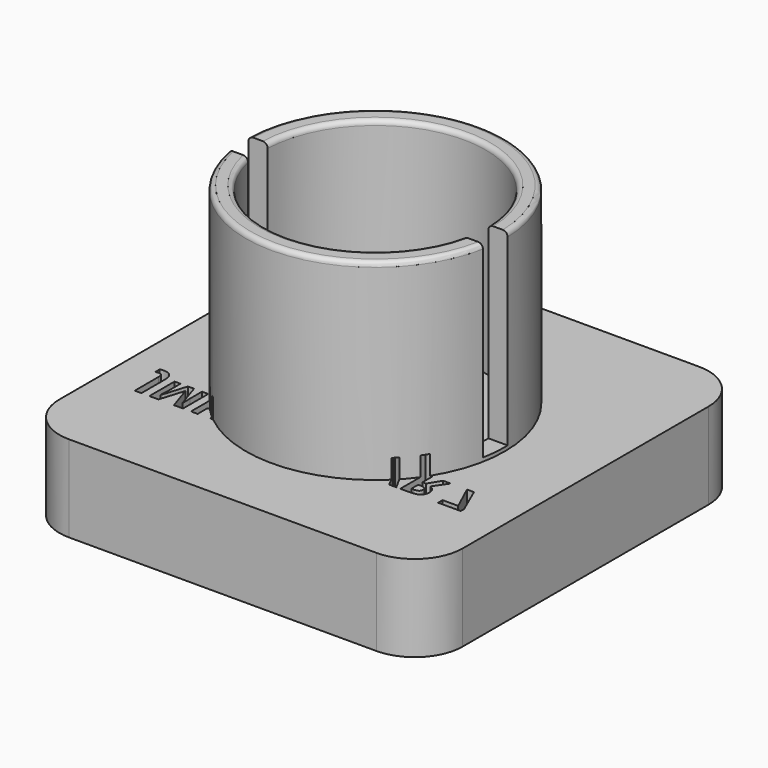
from build123d import *

# Parameters (mm, degrees)
F1_DEPTH      = 3
F2_R          = 13.5
F3_DEPTH      = 20
F4_T          = -2
F5_R          = 0.5
F6_TEXT_SIZE  = 4.5962860367
F7_DEPTH      = 5
F8_W          = 2.9094833881
F8_H          = 24.4396554772
F9_DEPTH      = 61.5
F10_DEPTH     = 6
F11_TEXT_SIZE = 3.6623448817
F12_DEPTH     = 7


# Not quite as in the source:
# - Text() gives the source's letters only with a copy of the font that has no kerning and outlines rounded to 1/6400 em; it was checked with that copy


with BuildPart() as f1:
    # F0 (on Top) → F1 (new body)
    with BuildSketch(Plane.XY):
        with BuildLine():
            ThreePointArc((0, 5), (1.4644660941, 1.4644660941), (5, 0))
            Line((5, 0), (37, 0))
            ThreePointArc((37, 0), (40.5355339059, 1.4644660941), (42, 5))
            Line((42, 5), (42, 37))
            ThreePointArc((42, 37), (40.5355339059, 40.5355339059), (37, 42))
            Line((37, 42), (5, 42))
            ThreePointArc((5, 42), (1.4644660941, 40.5355339059), (0, 37))
            Line((0, 37), (0, 5))
        make_face()
    extrude(amount=F1_DEPTH)

    # F2 (on face) → F3 (join)
    with BuildSketch(Plane.XY.offset(3)):
        with Locations((20.5, 20.5)):
            Circle(F2_R)
    extrude(amount=F3_DEPTH)

    # F4
    f4_openings = [f1.faces().sort_by_distance(p)[0] for p in [
        (20.5, 20.5, 23),
    ]]
    offset(amount=F4_T, openings=f4_openings, kind=Kind.INTERSECTION)

    # F5
    f5_edges = [f1.edges().sort_by_distance(p)[0] for p in [
        (9, 20.5, 23),
        (7, 20.5, 23),
    ]]
    fillet(f5_edges, radius=F5_R)

    # F6 (on face) → F7 (cut)
    with BuildSketch(Plane(origin=(0, 0, 0), x_dir=(1, 0, 0), z_dir=(0, 0, -1))):
        with Locations((3.4033681848, -13.3093259464)):
            Text('JMHS 2017 YR 7', F6_TEXT_SIZE, font='Open Sans', font_style=FontStyle.BOLD, text_align=(TextAlign.LEFT, TextAlign.BOTTOM))
    extrude(amount=-F7_DEPTH, mode=Mode.SUBTRACT)

    # F8 (on Right) → F9 (cut)
    with BuildSketch(Plane.YZ):
        with Locations((19.3965518847, 15.6142244814)):
            Rectangle(F8_W, F8_H)
    extrude(amount=F9_DEPTH, mode=Mode.SUBTRACT)

    # F10 (add): a face of the model
    f10_faces = [f1.faces().sort_by_distance(p)[0] for p in [
        (21.0498255374, 21.2729952215, 0),
    ]]
    extrude(f10_faces, amount=F10_DEPTH)

    # F11 (on face) → F12 (cut)
    with BuildSketch(Plane(origin=(0, 0, -6), x_dir=(1, 0, 0), z_dir=(0, 0, -1))):
        with Locations((3.3476579707, -30.9793796742)):
            Text('TEACHER:  MR KHAN', F11_TEXT_SIZE, font='Open Sans', text_align=(TextAlign.LEFT, TextAlign.BOTTOM))
    extrude(amount=-F12_DEPTH, mode=Mode.SUBTRACT)


solid = f1.part
